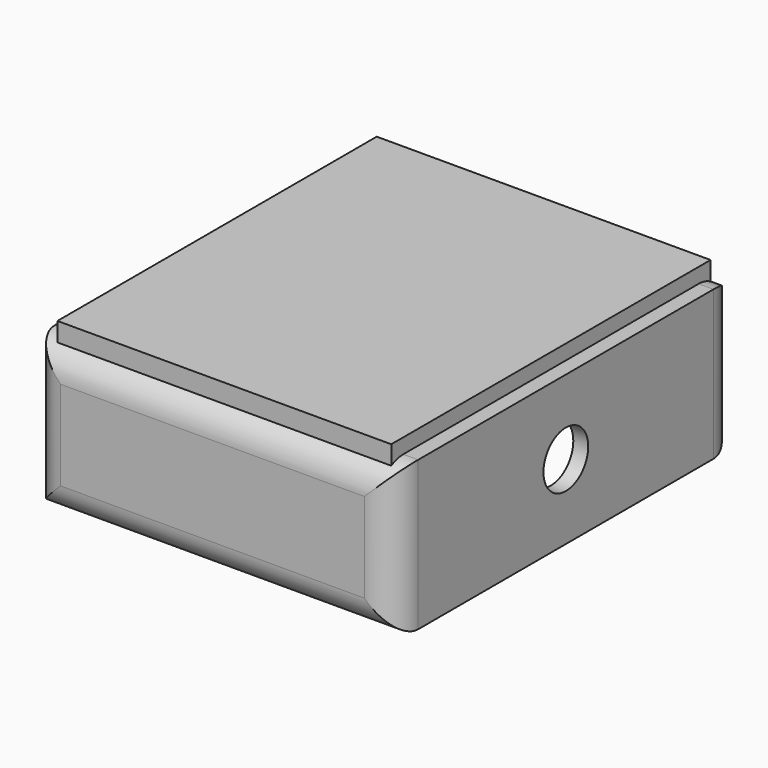
from build123d import *

# Parameters (mm, degrees)
F0_W         = 61.9125
F0_H         = 25.4
F1_DEPTH     = 73.025
F3_T         = -2.54
F4_W         = 56.8325
F4_H         = 67.945
F5_DEPTH     = 2.54
F6_T1_DEPTH  = 50.8
F6_T3_DEPTH  = 87.3125
F6_T8_DEPTH  = 87.3125
F6_T14_DEPTH = 87.3125
F6_T20_DEPTH = 87.3125
F6_T27_DEPTH = 87.3125
F6_T33_DEPTH = 87.3125
F7_T1_DEPTH  = 50.8
F7_T3_DEPTH  = 87.3125
F7_T8_DEPTH  = 87.3125
F7_T14_DEPTH = 87.3125
F7_T20_DEPTH = 87.3125
F7_T27_DEPTH = 87.3125
F7_T33_DEPTH = 87.3125
F2_R         = 4.7625
F8_DEPTH     = 61.9135
F10_DEPTH    = 19.05


# Not quite as in the source:
# - a fillet or chamfer that OpenCascade refuses, or shapes differently, is made with other operations: its cross-section is extruded or revolved along the edge and cut away or added


with BuildPart() as f1:
    # F0 (on Front) → F1 (new body)
    with BuildSketch(Plane.XZ):
        Rectangle(F0_W, F0_H)
    extrude(amount=F1_DEPTH)

    # F3
    f3_openings = [f1.faces().sort_by_distance(p)[0] for p in [
        (0, -36.5125, -12.7),
    ]]
    offset(amount=F3_T, openings=f3_openings)

    # F4 (on face) → F5 (join)
    with BuildSketch(Plane.XY.offset(12.7)):
        with Locations((0, -36.5125)):
            Rectangle(F4_W, F4_H)
    extrude(amount=F5_DEPTH)

    # F6: fillet of radius 5.08 on 4 edges, made by hand

    # F6_s2 → F6_t1 (cut)
    with BuildSketch(Plane.XY.offset(-25.4)):
        with BuildLine():
            ThreePointArc((-25.87625, 0), (-29.4683524484, -1.4878975516), (-30.95625, -5.08))
            Line((-30.95625, -5.08), (-30.95625, 0))
            Line((-30.95625, 0), (-25.87625, 0))
        make_face()
        with BuildLine():
            ThreePointArc((30.95625, -5.08), (29.4683524484, -1.4878975516), (25.87625, 0))
            Line((25.87625, 0), (30.95625, 0))
            Line((30.95625, 0), (30.95625, -5.08))
        make_face()
    extrude(amount=F6_T1_DEPTH, mode=Mode.SUBTRACT)

    # F6_s4 → F6_t3 (cut)
    with BuildSketch(Plane.YZ.offset(-43.65625)):
        with BuildLine():
            ThreePointArc((0, -7.62), (-1.4878975516, -11.2121024484), (-5.08, -12.7))
            Line((-5.08, -12.7), (0, -12.7))
            Line((0, -12.7), (0, -7.62))
        make_face()
    extrude(amount=F6_T3_DEPTH, mode=Mode.SUBTRACT)


with BuildPart() as f6_tool6:
    # F6_s7 → F6_t8 (new body)
    with BuildSketch(Plane.YZ.offset(43.65625)):
        with BuildLine():
            ThreePointArc((-5.08, 12.7), (-1.4878975516, 11.2121024484), (0, 7.62))
            Line((0, 7.62), (0, 12.7))
            Line((0, 12.7), (-5.08, 12.7))
        make_face()
    extrude(amount=-F6_T8_DEPTH)

    split(bisect_by=Plane.XZ.offset(2.54), keep=Keep.TOP)

    split(bisect_by=Plane.YZ.offset(28.41625), keep=Keep.TOP)


with BuildPart() as f1_1:
    add(f1.part)

    # F6_t5: cut F6_tool6
    add(f6_tool6.part, mode=Mode.SUBTRACT)


with BuildPart() as f6_tool12:
    # F6_s13 → F6_t14 (new body)
    with BuildSketch(Plane.YZ.offset(43.65625)):
        with BuildLine():
            ThreePointArc((-5.08, 12.7), (-1.4878975516, 11.2121024484), (0, 7.62))
            Line((0, 7.62), (0, 12.7))
            Line((0, 12.7), (-5.08, 12.7))
        make_face()
    extrude(amount=-F6_T14_DEPTH)

    split(bisect_by=Plane.XZ.offset(2.54), keep=Keep.BOTTOM)

    split(bisect_by=Plane.YZ.offset(28.41625), keep=Keep.TOP)


with BuildPart() as f1_2:
    add(f1_1.part)

    # F6_t11: cut F6_tool12
    add(f6_tool12.part, mode=Mode.SUBTRACT)


with BuildPart() as f6_tool18:
    # F6_s19 → F6_t20 (new body)
    with BuildSketch(Plane.YZ.offset(43.65625)):
        with BuildLine():
            ThreePointArc((-5.08, 12.7), (-1.4878975516, 11.2121024484), (0, 7.62))
            Line((0, 7.62), (0, 12.7))
            Line((0, 12.7), (-5.08, 12.7))
        make_face()
    extrude(amount=-F6_T20_DEPTH)

    split(bisect_by=Plane.YZ.offset(-28.41625), keep=Keep.TOP)

    split(bisect_by=Plane.XZ.offset(2.54), keep=Keep.BOTTOM)

    split(bisect_by=Plane.YZ.offset(28.41625), keep=Keep.BOTTOM)


with BuildPart() as f1_3:
    add(f1_2.part)

    # F6_t17: cut F6_tool18
    add(f6_tool18.part, mode=Mode.SUBTRACT)


with BuildPart() as f6_tool25:
    # F6_s26 → F6_t27 (new body)
    with BuildSketch(Plane.YZ.offset(43.65625)):
        with BuildLine():
            ThreePointArc((-5.08, 12.7), (-1.4878975516, 11.2121024484), (0, 7.62))
            Line((0, 7.62), (0, 12.7))
            Line((0, 12.7), (-5.08, 12.7))
        make_face()
    extrude(amount=-F6_T27_DEPTH)

    split(bisect_by=Plane.YZ.offset(-28.41625), keep=Keep.BOTTOM)

    split(bisect_by=Plane.XZ.offset(2.54), keep=Keep.TOP)


with BuildPart() as f1_4:
    add(f1_3.part)

    # F6_t24: cut F6_tool25
    add(f6_tool25.part, mode=Mode.SUBTRACT)


with BuildPart() as f6_tool31:
    # F6_s32 → F6_t33 (new body)
    with BuildSketch(Plane.YZ.offset(43.65625)):
        with BuildLine():
            ThreePointArc((-5.08, 12.7), (-1.4878975516, 11.2121024484), (0, 7.62))
            Line((0, 7.62), (0, 12.7))
            Line((0, 12.7), (-5.08, 12.7))
        make_face()
    extrude(amount=-F6_T33_DEPTH)

    split(bisect_by=Plane.YZ.offset(-28.41625), keep=Keep.BOTTOM)

    split(bisect_by=Plane.XZ.offset(2.54), keep=Keep.BOTTOM)


with BuildPart() as f1_5:
    add(f1_4.part)

    # F6_t30: cut F6_tool31
    add(f6_tool31.part, mode=Mode.SUBTRACT)

    # F7: fillet of radius 5.08 on 4 edges, made by hand

    # F7_s2 → F7_t1 (cut)
    with BuildSketch(Plane.XY.offset(-25.4)):
        with BuildLine():
            ThreePointArc((-25.87625, -73.025), (-29.4683524484, -71.5371024484), (-30.95625, -67.945))
            Line((-30.95625, -67.945), (-30.95625, -73.025))
            Line((-30.95625, -73.025), (-25.87625, -73.025))
        make_face()
        with BuildLine():
            ThreePointArc((30.95625, -67.945), (29.4683524484, -71.5371024484), (25.87625, -73.025))
            Line((25.87625, -73.025), (30.95625, -73.025))
            Line((30.95625, -73.025), (30.95625, -67.945))
        make_face()
    extrude(amount=F7_T1_DEPTH, mode=Mode.SUBTRACT)

    # F7_s4 → F7_t3 (cut)
    with BuildSketch(Plane.YZ.offset(-43.65625)):
        with BuildLine():
            ThreePointArc((-67.945, -12.7), (-71.5371024484, -11.2121024484), (-73.025, -7.62))
            Line((-73.025, -7.62), (-73.025, -12.7))
            Line((-73.025, -12.7), (-67.945, -12.7))
        make_face()
    extrude(amount=F7_T3_DEPTH, mode=Mode.SUBTRACT)


with BuildPart() as f7_tool6:
    # F7_s7 → F7_t8 (new body)
    with BuildSketch(Plane.YZ.offset(43.65625)):
        with BuildLine():
            ThreePointArc((-67.945, 12.7), (-71.5371024484, 11.2121024484), (-73.025, 7.62))
            Line((-73.025, 7.62), (-73.025, 12.7))
            Line((-73.025, 12.7), (-67.945, 12.7))
        make_face()
    extrude(amount=-F7_T8_DEPTH)

    split(bisect_by=Plane.YZ.offset(28.41625), keep=Keep.TOP)

    split(bisect_by=Plane.XZ.offset(70.485), keep=Keep.BOTTOM)


with BuildPart() as f1_6:
    add(f1_5.part)

    # F7_t5: cut F7_tool6
    add(f7_tool6.part, mode=Mode.SUBTRACT)


with BuildPart() as f7_tool12:
    # F7_s13 → F7_t14 (new body)
    with BuildSketch(Plane.YZ.offset(43.65625)):
        with BuildLine():
            ThreePointArc((-67.945, 12.7), (-71.5371024484, 11.2121024484), (-73.025, 7.62))
            Line((-73.025, 7.62), (-73.025, 12.7))
            Line((-73.025, 12.7), (-67.945, 12.7))
        make_face()
    extrude(amount=-F7_T14_DEPTH)

    split(bisect_by=Plane.YZ.offset(28.41625), keep=Keep.TOP)

    split(bisect_by=Plane.XZ.offset(70.485), keep=Keep.TOP)


with BuildPart() as f1_7:
    add(f1_6.part)

    # F7_t11: cut F7_tool12
    add(f7_tool12.part, mode=Mode.SUBTRACT)


with BuildPart() as f7_tool18:
    # F7_s19 → F7_t20 (new body)
    with BuildSketch(Plane.YZ.offset(43.65625)):
        with BuildLine():
            ThreePointArc((-67.945, 12.7), (-71.5371024484, 11.2121024484), (-73.025, 7.62))
            Line((-73.025, 7.62), (-73.025, 12.7))
            Line((-73.025, 12.7), (-67.945, 12.7))
        make_face()
    extrude(amount=-F7_T20_DEPTH)

    split(bisect_by=Plane.YZ.offset(28.41625), keep=Keep.BOTTOM)

    split(bisect_by=Plane.XZ.offset(70.485), keep=Keep.TOP)

    split(bisect_by=Plane.YZ.offset(-28.41625), keep=Keep.TOP)


with BuildPart() as f1_8:
    add(f1_7.part)

    # F7_t17: cut F7_tool18
    add(f7_tool18.part, mode=Mode.SUBTRACT)


with BuildPart() as f7_tool25:
    # F7_s26 → F7_t27 (new body)
    with BuildSketch(Plane.YZ.offset(43.65625)):
        with BuildLine():
            ThreePointArc((-67.945, 12.7), (-71.5371024484, 11.2121024484), (-73.025, 7.62))
            Line((-73.025, 7.62), (-73.025, 12.7))
            Line((-73.025, 12.7), (-67.945, 12.7))
        make_face()
    extrude(amount=-F7_T27_DEPTH)

    split(bisect_by=Plane.XZ.offset(70.485), keep=Keep.BOTTOM)

    split(bisect_by=Plane.YZ.offset(-28.41625), keep=Keep.BOTTOM)


with BuildPart() as f1_9:
    add(f1_8.part)

    # F7_t24: cut F7_tool25
    add(f7_tool25.part, mode=Mode.SUBTRACT)


with BuildPart() as f7_tool31:
    # F7_s32 → F7_t33 (new body)
    with BuildSketch(Plane.YZ.offset(43.65625)):
        with BuildLine():
            ThreePointArc((-67.945, 12.7), (-71.5371024484, 11.2121024484), (-73.025, 7.62))
            Line((-73.025, 7.62), (-73.025, 12.7))
            Line((-73.025, 12.7), (-67.945, 12.7))
        make_face()
    extrude(amount=-F7_T33_DEPTH)

    split(bisect_by=Plane.XZ.offset(70.485), keep=Keep.TOP)

    split(bisect_by=Plane.YZ.offset(-28.41625), keep=Keep.BOTTOM)


with BuildPart() as f1_10:
    add(f1_9.part)

    # F7_t30: cut F7_tool31
    add(f7_tool31.part, mode=Mode.SUBTRACT)

    # F2 (on face) → F8 (cut, through all)
    with BuildSketch(Plane.YZ.offset(30.95625)):
        with Locations((-36.5125, 0)):
            Circle(F2_R)
    extrude(amount=-F8_DEPTH, mode=Mode.SUBTRACT)

    # F9 (on face) → F10 (join)
    with BuildSketch(Plane(origin=(0, 0, 10.16), x_dir=(1, 0, 0), z_dir=(0, 0, -1))):
        Polygon((-3.175, 61.9125), (3.175, 61.9125), (3.175, 59.2770799994), (6.35, 59.3725), (6.35, 61.9125), (6.35, 70.485), (0, 70.485), (-6.35, 70.485), (-6.35, 61.9125), (-6.35, 59.3725), (-3.175, 59.3725), align=None)
        Polygon((3.175, 13.6525), (3.175, 11.1125), (-3.175, 11.1125), (-3.175, 13.6525), (-6.35, 13.6525), (-6.35, 11.1125), (-6.35, 2.54), (6.35, 2.54), (6.35, 11.1125), (6.35, 13.6525), align=None)
    extrude(amount=F10_DEPTH)


solid = f1_10.part
